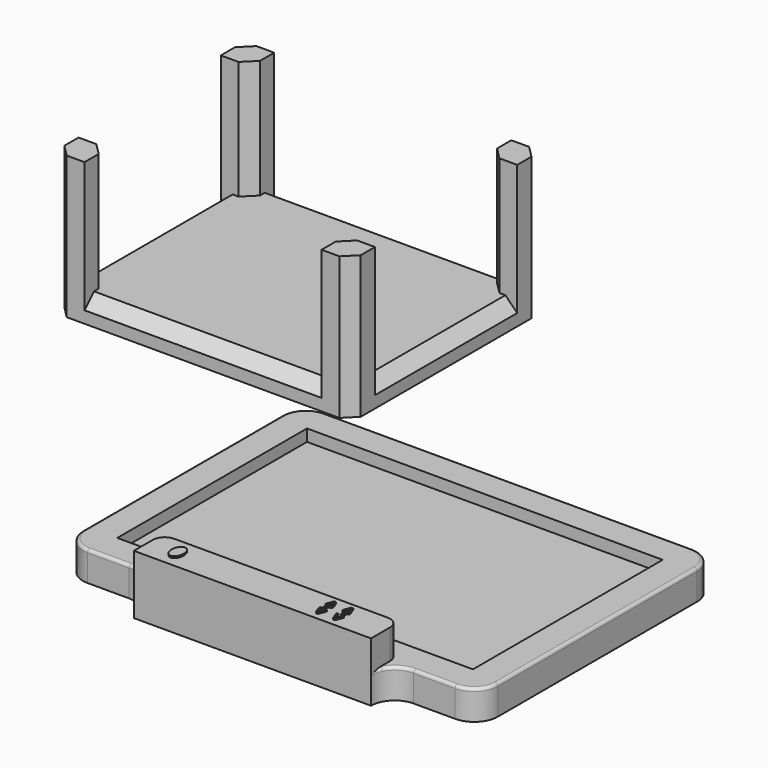
from build123d import *

# Parameters (mm, degrees)
F0_W          = 88.9
F0_H          = 63.5
F1_DEPTH      = 6.35
F2_W          = 76.2
F2_H          = 50.8
F3_DEPTH      = 2.54
F5_DEPTH      = 5.08
F6_DEPTH      = 2.54
F7_R          = 5.07999
F8_R          = 2.54
F10_DEPTH     = 0.381
F12_DEPTH     = 0.254
F13_TEXT_SIZE = 1.5415140206
F14_DEPTH     = 0.254
F15_R         = 0.635
F16_W         = 63.5
F16_H         = 50.8
F17_DEPTH     = 5.08
F18_W         = 6.35
F18_H         = 6.35
F19_DEPTH     = 25.4
F20_SIZE      = 2.54


# Not quite as in the source:
# - a fillet or chamfer is up to 0.001 mm smaller than in the source, because OpenCascade refuses the exact size
# - Text() gives the source's letters only with a copy of the font that has no kerning and outlines rounded to 1/6400 em; it was checked with that copy


with BuildPart() as f1:
    # F0 (on Top) → F1 (new body)
    with BuildSketch(Plane.XY):
        Rectangle(F0_W, F0_H)
    extrude(amount=F1_DEPTH)

    # F2 (on face) → F3 (cut)
    with BuildSketch(Plane.XY.offset(6.35)):
        Rectangle(F2_W, F2_H)
    extrude(amount=-F3_DEPTH, mode=Mode.SUBTRACT)

    # F4 (on face) → F5 (join)
    with BuildSketch(Plane.XZ.offset(31.75)):
        Polygon((0, 0), (25.4, 0), (25.4, 12.7), (-25.4, 12.7), (-25.4, 0), align=None)
    extrude(amount=F5_DEPTH)

    # F6 (add): a face of the model
    f6_faces = [f1.faces().sort_by_distance(p)[0] for p in [
        (0, -31.75, 9.525),
    ]]
    extrude(f6_faces, amount=F6_DEPTH)

    # F7 (radius 5.08 in the source; OpenCascade refuses exactly that, so slightly less here)
    f7_edges = [f1.edges().sort_by_distance(p)[0] for p in [
        (25.4, -31.75, 3.175),
        (-25.4, -31.75, 3.175),
        (44.45, 31.75, 3.175),
        (44.45, -31.75, 3.175),
        (-44.45, -31.75, 3.175),
        (-44.45, 31.75, 3.175),
    ]]
    fillet(f7_edges, radius=F7_R)

    # F8
    f8_edges = [f1.edges().sort_by_distance(p)[0] for p in [
        (-25.4, -29.21, 9.525),
        (25.4, -29.21, 9.525),
    ]]
    fillet(f8_edges, radius=F8_R)

    # F9 (on face) → F10 (join)
    with BuildSketch(Plane.XY.offset(12.7)):
        with BuildLine():
            add(Edge.make_bspline(
                [(-19.9966021105, -34.29), (-18.6904844022, -36.4804259867), (-17.8906539199, -33.7977129933), (-17.0908234377, -31.115), (-19.05, -31.115)],
                knots=[2.300523983, 2.300523983, 2.300523983, 4.2918546451, 4.2918546451, 6.2831853072, 6.2831853072, 6.2831853072], degree=2, weights=[1, 0.5439447166, 1, 0.5439447166, 1]))
            add(Edge.make_bspline(
                [(-19.05, -31.115), (-21.8898063314, -31.115), (-19.9966021105, -34.29)],
                knots=[0, 0, 0, 2.300523983, 2.300523983, 2.300523983], degree=2, weights=[1, 0.4082482905, 1]))
        make_face()
    extrude(amount=F10_DEPTH)

    # F11 (on face) → F12 (join)
    with BuildSketch(Plane.XY.offset(12.7)):
        Polygon((13.558951327, -32.1875824289), (12.9485117749, -30.5782417914), (12.5045557369, -30.5782417914), (11.8941161848, -32.1875824289), (12.1715887085, -32.4650549526), (12.7265337559, -30.8002198104), (13.2814788033, -32.4650549526), align=None)
        Polygon((13.558951327, -33.8524175711), (13.2814788033, -33.5749450474), (12.7265337559, -35.2397801896), (12.1715887085, -33.5749450474), (11.8941161848, -33.8524175711), (12.5045557369, -35.4617582086), (12.9485117749, -35.4617582086), align=None)
        Polygon((15.8214788033, -32.4650549526), (16.3764238507, -30.8002198104), (16.9313688981, -32.4650549526), (17.2088414218, -32.1875824289), (16.5984018697, -30.5782417914), (16.1544458317, -30.5782417914), (15.5440062796, -32.1875824289), align=None)
        Polygon((17.2088414218, -33.8524175711), (16.9313688981, -33.5749450474), (16.3764238507, -35.2397801896), (15.8214788033, -33.5749450474), (15.5440062796, -33.8524175711), (16.1544458317, -35.4617582086), (16.5984018697, -35.4617582086), align=None)
        with BuildLine():
            add(Edge.make_bspline(
                [(12.9833374244, -32.4650549526), (13.0925580635, -32.4786865168), (13.1814148597, -32.5219587856)],
                knots=[0.3150184776, 0.3150184776, 0.3150184776, 1, 1, 1], degree=2))
            Line((12.9833374244, -32.4650549526), (12.7845310367, -32.4650549526))
            add(Edge.make_bspline(
                [(12.5956188329, -32.528107293), (12.6796699423, -32.4796324807), (12.7845310367, -32.4650549526)],
                knots=[0, 0, 0, 0.6992762354, 0.6992762354, 0.6992762354], degree=2))
            add(Edge.make_bspline(
                [(12.4117664064, -32.725462324), (12.4754215416, -32.5974286997), (12.5956188329, -32.528107293)],
                knots=[0, 0, 0, 1, 1, 1], degree=2))
            add(Edge.make_bspline(
                [(12.3481112711, -33.0237252115), (12.3481112711, -32.8534959483), (12.4117664064, -32.725462324)],
                knots=[0, 0, 0, 1, 1, 1], degree=2))
            add(Edge.make_bspline(
                [(12.4803644593, -33.4435115389), (12.3481112711, -33.2957062438), (12.3481112711, -33.0237252115)],
                knots=[0, 0, 0, 1, 1, 1], degree=2))
            add(Edge.make_bspline(
                [(12.7062646704, -33.5749450474), (12.5686017875, -33.5421249978), (12.4803644593, -33.4435115389)],
                knots=[0.3328151143, 0.3328151143, 0.3328151143, 1, 1, 1], degree=2))
            Line((12.7062646704, -33.5749450474), (13.0426146558, -33.5749450474))
            add(Edge.make_bspline(
                [(13.138495867, -33.5481567233), (13.0945039433, -33.5647347325), (13.0426146558, -33.5749450474)],
                knots=[0, 0, 0, 0.3841048806, 0.3841048806, 0.3841048806], degree=2))
            Line((13.138495867, -33.5481567233), (13.138495867, -33.4360368829))
            add(Edge.make_bspline(
                [(12.8754361982, -33.477509168), (12.9906905719, -33.477509168), (13.138495867, -33.4360368829)],
                knots=[0, 0, 0, 1, 1, 1], degree=2))
            add(Edge.make_bspline(
                [(12.5864563513, -33.359481938), (12.6878464436, -33.477509168), (12.8754361982, -33.477509168)],
                knots=[0, 0, 0, 1, 1, 1], degree=2))
            add(Edge.make_bspline(
                [(12.4850662591, -33.025413037), (12.4850662591, -33.2414547081), (12.5864563513, -33.359481938)],
                knots=[0, 0, 0, 1, 1, 1], degree=2))
            add(Edge.make_bspline(
                [(12.5901936794, -32.6942375512), (12.4850662591, -32.8151581964), (12.4850662591, -33.025413037)],
                knots=[0, 0, 0, 1, 1, 1], degree=2))
            add(Edge.make_bspline(
                [(12.8768829059, -32.5733169061), (12.6953210997, -32.5733169061), (12.5901936794, -32.6942375512)],
                knots=[0, 0, 0, 1, 1, 1], degree=2))
            add(Edge.make_bspline(
                [(13.1271633239, -32.6319085647), (13.0020231149, -32.5733169061), (12.8768829059, -32.5733169061)],
                knots=[0, 0, 0, 1, 1, 1], degree=2))
            Line((13.1271633239, -32.6319085647), (13.1814148597, -32.5219587856))
        make_face()
    extrude(amount=F12_DEPTH)

    # F13 (on face) → F14 (join)
    with BuildSketch(Plane.XY.offset(12.7)):
        with Locations((15.9681495279, -33.5749450474)):
            Text('V', F13_TEXT_SIZE, font='Open Sans', text_align=(TextAlign.LEFT, TextAlign.BOTTOM))
    extrude(amount=F14_DEPTH)

    # F15
    f15_edges = [f1.edges().sort_by_distance(p)[0] for p in [
        (0, 31.75, 6.35),
        (-44.45, 0, 6.35),
        (44.45, 0, 6.35),
        (-34.925, -31.75, 6.35),
        (34.925, -31.75, 6.35),
        (42.962105, -30.262105, 6.35),
        (42.962105, 30.262105, 6.35),
        (-42.962105, 30.262105, 6.35),
        (-42.962105, -30.262105, 6.35),
    ]]
    fillet(f15_edges, radius=F15_R)


with BuildPart() as f17:
    # F16 (on Top) → F17 (new body)
    with BuildSketch(Plane.XY):
        with Locations((-73.0734094977, 66.6826953449)):
            Rectangle(F16_W, F16_H)
    extrude(amount=F17_DEPTH)

    # F18 (on face) → F19 (join)
    with BuildSketch(Plane.XY.offset(5.08)):
        with Locations((-101.6484094977, 88.9076953449)):
            Rectangle(F18_W, F18_H)
        with Locations((-44.4984094977, 88.9076953449)):
            Rectangle(F18_W, F18_H)
        with Locations((-44.4984094977, 44.4576953449)):
            Rectangle(F18_W, F18_H)
        with Locations((-101.6484094977, 44.4576953449)):
            Rectangle(F18_W, F18_H)
    extrude(amount=F19_DEPTH)

    # F20
    f20_edges = [f17.edges().sort_by_distance(p)[0] for p in [
        (-41.323409, 41.282695, 15.24),
        (-41.323409, 92.082695, 15.24),
        (-104.823409, 41.282695, 15.24),
        (-104.823409, 92.082695, 15.24),
        (-73.073409, 92.082695, 5.08),
        (-41.323409, 66.682695, 5.08),
        (-73.073409, 41.282695, 5.08),
        (-104.823409, 66.682695, 5.08),
        (-98.473409, 47.632695, 17.78),
        (-98.473409, 85.732695, 17.78),
        (-47.673409, 85.732695, 17.78),
        (-47.673409, 47.632695, 17.78),
    ]]
    chamfer(f20_edges, length=F20_SIZE)


solid = Compound([f1.part, f17.part])
